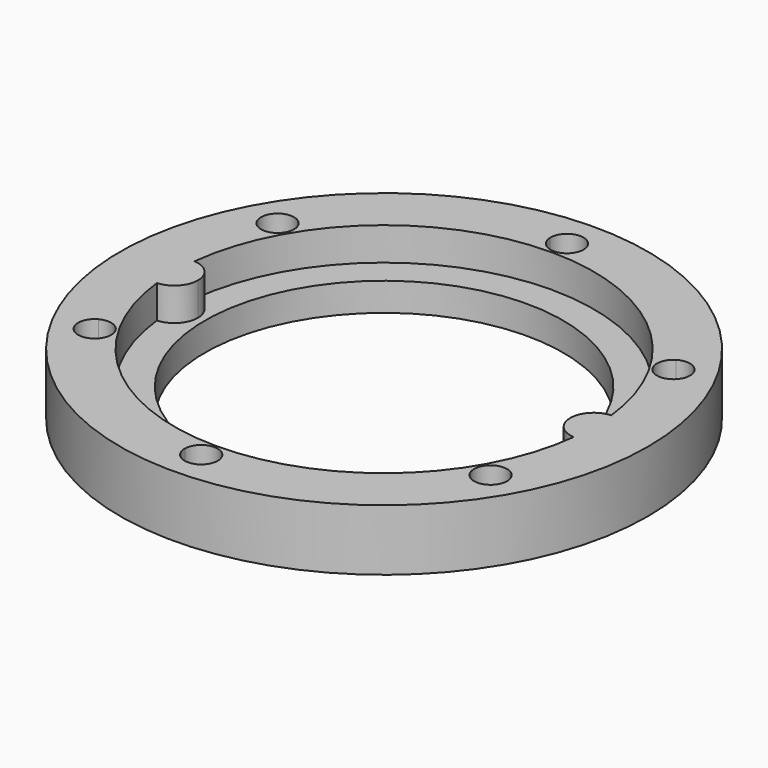
from build123d import *

# Parameters (mm, degrees)
F0_R     = 28
F1_DEPTH = 3.5
F0_R_2   = 19
F2_DEPTH = 3


with BuildPart() as f1:
    # F0 (on Top) → F1 (new body)
    with BuildSketch(Plane.XY):
        Circle(F0_R)
        with BuildLine():
            ThreePointArc((21.8208616615, 10.5788702775), (23.4473621908, 6.1873828305), (24.1994382022, 1.5651487775))
            ThreePointArc((24.1994382022, 1.5651487775), (24.6083464022, 0.8295795605), (24.75, 0))
            ThreePointArc((24.75, 0), (24.6083464022, -0.8295795605), (24.1994382022, -1.5651487775))
            ThreePointArc((24.1994382022, -1.5651487775), (23.4473621908, -6.1873828305), (21.8208616615, -10.5788702775))
            ThreePointArc((21.8208616615, -10.5788702775), (22.5006251005, -11.222795709), (22.7511160418, -12.125))
            ThreePointArc((22.7511160418, -12.125), (21.8486268344, -13.6560863648), (20.0720012344, -13.6079853926))
            ThreePointArc((20.0720012344, -13.6079853926), (12.125, -21.0011160418), (1.7488604271, -24.1868556701))
            ThreePointArc((1.7488604271, -24.1868556701), (1.7497150836, -24.218422694), (1.75, -24.25))
            ThreePointArc((1.75, -24.25), (-0.031577306, -25.9997150836), (-1.7488604271, -24.1868556701))
            ThreePointArc((-1.7488604271, -24.1868556701), (-12.125, -21.0011160418), (-20.0720012344, -13.6079853926))
            ThreePointArc((-20.0720012344, -13.6079853926), (-22.5166604984, -13), (-21.8208616615, -10.5788702775))
            ThreePointArc((-21.8208616615, -10.5788702775), (-23.4473621908, -6.1873828305), (-24.1994382022, -1.5651487775))
            ThreePointArc((-24.1994382022, -1.5651487775), (-24.75, 0), (-24.1994382022, 1.5651487775))
            ThreePointArc((-24.1994382022, 1.5651487775), (-23.4473621908, 6.1873828305), (-21.8208616615, 10.5788702775))
            ThreePointArc((-21.8208616615, 10.5788702775), (-22.5166604984, 13), (-20.0720012344, 13.6079853926))
            ThreePointArc((-20.0720012344, 13.6079853926), (-12.125, 21.0011160418), (-1.7488604271, 24.1868556701))
            ThreePointArc((-1.7488604271, 24.1868556701), (-0.031577306, 25.9997150836), (1.75, 24.25))
            ThreePointArc((1.75, 24.25), (1.7497150836, 24.218422694), (1.7488604271, 24.1868556701))
            ThreePointArc((1.7488604271, 24.1868556701), (12.125, 21.0011160418), (20.0720012344, 13.6079853926))
            ThreePointArc((20.0720012344, 13.6079853926), (21.8486268344, 13.6560863648), (22.7511160418, 12.125))
            ThreePointArc((22.7511160418, 12.125), (22.5006251005, 11.222795709), (21.8208616615, 10.5788702775))
        make_face(mode=Mode.SUBTRACT)
        with BuildLine():
            ThreePointArc((22.1095505618, 2.4960516732), (23.267229147, 2.2836910611), (24.1994382022, 1.5651487775))
            ThreePointArc((24.1994382022, 1.5651487775), (23.4473621908, 6.1873828305), (21.8208616615, 10.5788702775))
            ThreePointArc((21.8208616615, 10.5788702775), (19.4855715851, 11.25), (20.0720012344, 13.6079853926))
            ThreePointArc((20.0720012344, 13.6079853926), (12.125, 21.0011160418), (1.7488604271, 24.1868556701))
            ThreePointArc((1.7488604271, 24.1868556701), (0, 22.5), (-1.7488604271, 24.1868556701))
            ThreePointArc((-1.7488604271, 24.1868556701), (-12.125, 21.0011160418), (-20.0720012344, 13.6079853926))
            ThreePointArc((-20.0720012344, 13.6079853926), (-19.470029677, 12.9725107926), (-19.2511160418, 12.125))
            ThreePointArc((-19.2511160418, 12.125), (-20.0989117508, 10.6254909412), (-21.8208616615, 10.5788702775))
            ThreePointArc((-21.8208616615, 10.5788702775), (-23.4473621908, 6.1873828305), (-24.1994382022, 1.5651487775))
            ThreePointArc((-24.1994382022, 1.5651487775), (-23.267229147, 2.2836910611), (-22.1095505618, 2.4960516732))
            ThreePointArc((-22.1095505618, 2.4960516732), (0, 22.25), (22.1095505618, 2.4960516732))
        make_face()
        with BuildLine():
            ThreePointArc((21.8208616615, -10.5788702775), (23.4473621908, -6.1873828305), (24.1994382022, -1.5651487775))
            ThreePointArc((24.1994382022, -1.5651487775), (23.267229147, -2.2836910611), (22.1095505618, -2.4960516732))
            ThreePointArc((22.1095505618, -2.4960516732), (0, -22.25), (-22.1095505618, -2.4960516732))
            ThreePointArc((-22.1095505618, -2.4960516732), (-23.267229147, -2.2836910611), (-24.1994382022, -1.5651487775))
            ThreePointArc((-24.1994382022, -1.5651487775), (-23.4473621908, -6.1873828305), (-21.8208616615, -10.5788702775))
            ThreePointArc((-21.8208616615, -10.5788702775), (-20.0989117508, -10.6254909412), (-19.2511160418, -12.125))
            ThreePointArc((-19.2511160418, -12.125), (-19.470029677, -12.9725107926), (-20.0720012344, -13.6079853926))
            ThreePointArc((-20.0720012344, -13.6079853926), (-12.125, -21.0011160418), (-1.7488604271, -24.1868556701))
            ThreePointArc((-1.7488604271, -24.1868556701), (0, -22.5), (1.7488604271, -24.1868556701))
            ThreePointArc((1.7488604271, -24.1868556701), (12.125, -21.0011160418), (20.0720012344, -13.6079853926))
            ThreePointArc((20.0720012344, -13.6079853926), (19.4855715851, -11.25), (21.8208616615, -10.5788702775))
        make_face()
        with BuildLine():
            ThreePointArc((22.25, 0), (22.2148598915, 1.25), (22.1095505618, 2.4960516732))
            ThreePointArc((22.1095505618, 2.4960516732), (19.75, 0), (22.1095505618, -2.4960516732))
            ThreePointArc((22.1095505618, -2.4960516732), (22.2148598915, -1.25), (22.25, 0))
        make_face()
        with BuildLine():
            ThreePointArc((-19.75, 0), (-20.4332551644, 1.7173928503), (-22.1095505618, 2.4960516732))
            ThreePointArc((-22.1095505618, 2.4960516732), (-22.25, 0), (-22.1095505618, -2.4960516732))
            ThreePointArc((-22.1095505618, -2.4960516732), (-20.4332551644, -1.7173928503), (-19.75, 0))
        make_face()
        with BuildLine():
            ThreePointArc((24.1994382022, -1.5651487775), (24.2373562544, -0.7829826293), (24.25, 0))
            ThreePointArc((24.25, 0), (24.2373562544, 0.7829826293), (24.1994382022, 1.5651487775))
            ThreePointArc((24.1994382022, 1.5651487775), (23.267229147, 2.2836910611), (22.1095505618, 2.4960516732))
            ThreePointArc((22.1095505618, 2.4960516732), (22.2148598915, 1.25), (22.25, 0))
            ThreePointArc((22.25, 0), (22.2148598915, -1.25), (22.1095505618, -2.4960516732))
            ThreePointArc((22.1095505618, -2.4960516732), (23.267229147, -2.2836910611), (24.1994382022, -1.5651487775))
        make_face()
        with BuildLine():
            ThreePointArc((-22.1095505618, -2.4960516732), (-22.25, 0), (-22.1095505618, 2.4960516732))
            ThreePointArc((-22.1095505618, 2.4960516732), (-23.267229147, 2.2836910611), (-24.1994382022, 1.5651487775))
            ThreePointArc((-24.1994382022, 1.5651487775), (-24.25, 0), (-24.1994382022, -1.5651487775))
            ThreePointArc((-24.1994382022, -1.5651487775), (-23.267229147, -2.2836910611), (-22.1095505618, -2.4960516732))
        make_face()
        with BuildLine():
            ThreePointArc((24.1994382022, 1.5651487775), (24.2373562544, 0.7829826293), (24.25, 0))
            ThreePointArc((24.25, 0), (24.2373562544, -0.7829826293), (24.1994382022, -1.5651487775))
            ThreePointArc((24.1994382022, -1.5651487775), (24.6083464022, -0.8295795605), (24.75, 0))
            ThreePointArc((24.75, 0), (24.6083464022, 0.8295795605), (24.1994382022, 1.5651487775))
        make_face()
        with BuildLine():
            ThreePointArc((-24.1994382022, -1.5651487775), (-24.25, 0), (-24.1994382022, 1.5651487775))
            ThreePointArc((-24.1994382022, 1.5651487775), (-24.75, 0), (-24.1994382022, -1.5651487775))
        make_face()
    extrude(amount=F1_DEPTH)

    # F0 (on Top) → F2 (join)
    with BuildSketch(Plane.XY):
        Circle(F0_R)
        with BuildLine():
            ThreePointArc((21.8208616615, 10.5788702775), (23.4473621908, 6.1873828305), (24.1994382022, 1.5651487775))
            ThreePointArc((24.1994382022, 1.5651487775), (24.6083464022, 0.8295795605), (24.75, 0))
            ThreePointArc((24.75, 0), (24.6083464022, -0.8295795605), (24.1994382022, -1.5651487775))
            ThreePointArc((24.1994382022, -1.5651487775), (23.4473621908, -6.1873828305), (21.8208616615, -10.5788702775))
            ThreePointArc((21.8208616615, -10.5788702775), (22.5006251005, -11.222795709), (22.7511160418, -12.125))
            ThreePointArc((22.7511160418, -12.125), (21.8486268344, -13.6560863648), (20.0720012344, -13.6079853926))
            ThreePointArc((20.0720012344, -13.6079853926), (12.125, -21.0011160418), (1.7488604271, -24.1868556701))
            ThreePointArc((1.7488604271, -24.1868556701), (1.7497150836, -24.218422694), (1.75, -24.25))
            ThreePointArc((1.75, -24.25), (-0.031577306, -25.9997150836), (-1.7488604271, -24.1868556701))
            ThreePointArc((-1.7488604271, -24.1868556701), (-12.125, -21.0011160418), (-20.0720012344, -13.6079853926))
            ThreePointArc((-20.0720012344, -13.6079853926), (-22.5166604984, -13), (-21.8208616615, -10.5788702775))
            ThreePointArc((-21.8208616615, -10.5788702775), (-23.4473621908, -6.1873828305), (-24.1994382022, -1.5651487775))
            ThreePointArc((-24.1994382022, -1.5651487775), (-24.75, 0), (-24.1994382022, 1.5651487775))
            ThreePointArc((-24.1994382022, 1.5651487775), (-23.4473621908, 6.1873828305), (-21.8208616615, 10.5788702775))
            ThreePointArc((-21.8208616615, 10.5788702775), (-22.5166604984, 13), (-20.0720012344, 13.6079853926))
            ThreePointArc((-20.0720012344, 13.6079853926), (-12.125, 21.0011160418), (-1.7488604271, 24.1868556701))
            ThreePointArc((-1.7488604271, 24.1868556701), (-0.031577306, 25.9997150836), (1.75, 24.25))
            ThreePointArc((1.75, 24.25), (1.7497150836, 24.218422694), (1.7488604271, 24.1868556701))
            ThreePointArc((1.7488604271, 24.1868556701), (12.125, 21.0011160418), (20.0720012344, 13.6079853926))
            ThreePointArc((20.0720012344, 13.6079853926), (21.8486268344, 13.6560863648), (22.7511160418, 12.125))
            ThreePointArc((22.7511160418, 12.125), (22.5006251005, 11.222795709), (21.8208616615, 10.5788702775))
        make_face(mode=Mode.SUBTRACT)
        with BuildLine():
            ThreePointArc((22.1095505618, -2.4960516732), (19.75, 0), (22.1095505618, 2.4960516732))
            ThreePointArc((22.1095505618, 2.4960516732), (0, 22.25), (-22.1095505618, 2.4960516732))
            ThreePointArc((-22.1095505618, 2.4960516732), (-20.4332551644, 1.7173928503), (-19.75, 0))
            ThreePointArc((-19.75, 0), (-20.4332551644, -1.7173928503), (-22.1095505618, -2.4960516732))
            ThreePointArc((-22.1095505618, -2.4960516732), (0, -22.25), (22.1095505618, -2.4960516732))
        make_face()
        Circle(F0_R_2, mode=Mode.SUBTRACT)
        with BuildLine():
            ThreePointArc((22.1095505618, 2.4960516732), (23.267229147, 2.2836910611), (24.1994382022, 1.5651487775))
            ThreePointArc((24.1994382022, 1.5651487775), (23.4473621908, 6.1873828305), (21.8208616615, 10.5788702775))
            ThreePointArc((21.8208616615, 10.5788702775), (19.4855715851, 11.25), (20.0720012344, 13.6079853926))
            ThreePointArc((20.0720012344, 13.6079853926), (12.125, 21.0011160418), (1.7488604271, 24.1868556701))
            ThreePointArc((1.7488604271, 24.1868556701), (0, 22.5), (-1.7488604271, 24.1868556701))
            ThreePointArc((-1.7488604271, 24.1868556701), (-12.125, 21.0011160418), (-20.0720012344, 13.6079853926))
            ThreePointArc((-20.0720012344, 13.6079853926), (-19.470029677, 12.9725107926), (-19.2511160418, 12.125))
            ThreePointArc((-19.2511160418, 12.125), (-20.0989117508, 10.6254909412), (-21.8208616615, 10.5788702775))
            ThreePointArc((-21.8208616615, 10.5788702775), (-23.4473621908, 6.1873828305), (-24.1994382022, 1.5651487775))
            ThreePointArc((-24.1994382022, 1.5651487775), (-23.267229147, 2.2836910611), (-22.1095505618, 2.4960516732))
            ThreePointArc((-22.1095505618, 2.4960516732), (0, 22.25), (22.1095505618, 2.4960516732))
        make_face()
        with BuildLine():
            ThreePointArc((21.8208616615, -10.5788702775), (23.4473621908, -6.1873828305), (24.1994382022, -1.5651487775))
            ThreePointArc((24.1994382022, -1.5651487775), (23.267229147, -2.2836910611), (22.1095505618, -2.4960516732))
            ThreePointArc((22.1095505618, -2.4960516732), (0, -22.25), (-22.1095505618, -2.4960516732))
            ThreePointArc((-22.1095505618, -2.4960516732), (-23.267229147, -2.2836910611), (-24.1994382022, -1.5651487775))
            ThreePointArc((-24.1994382022, -1.5651487775), (-23.4473621908, -6.1873828305), (-21.8208616615, -10.5788702775))
            ThreePointArc((-21.8208616615, -10.5788702775), (-20.0989117508, -10.6254909412), (-19.2511160418, -12.125))
            ThreePointArc((-19.2511160418, -12.125), (-19.470029677, -12.9725107926), (-20.0720012344, -13.6079853926))
            ThreePointArc((-20.0720012344, -13.6079853926), (-12.125, -21.0011160418), (-1.7488604271, -24.1868556701))
            ThreePointArc((-1.7488604271, -24.1868556701), (0, -22.5), (1.7488604271, -24.1868556701))
            ThreePointArc((1.7488604271, -24.1868556701), (12.125, -21.0011160418), (20.0720012344, -13.6079853926))
            ThreePointArc((20.0720012344, -13.6079853926), (19.4855715851, -11.25), (21.8208616615, -10.5788702775))
        make_face()
        with BuildLine():
            ThreePointArc((22.25, 0), (22.2148598915, 1.25), (22.1095505618, 2.4960516732))
            ThreePointArc((22.1095505618, 2.4960516732), (19.75, 0), (22.1095505618, -2.4960516732))
            ThreePointArc((22.1095505618, -2.4960516732), (22.2148598915, -1.25), (22.25, 0))
        make_face()
        with BuildLine():
            ThreePointArc((-19.75, 0), (-20.4332551644, 1.7173928503), (-22.1095505618, 2.4960516732))
            ThreePointArc((-22.1095505618, 2.4960516732), (-22.25, 0), (-22.1095505618, -2.4960516732))
            ThreePointArc((-22.1095505618, -2.4960516732), (-20.4332551644, -1.7173928503), (-19.75, 0))
        make_face()
        with BuildLine():
            ThreePointArc((24.1994382022, -1.5651487775), (24.2373562544, -0.7829826293), (24.25, 0))
            ThreePointArc((24.25, 0), (24.2373562544, 0.7829826293), (24.1994382022, 1.5651487775))
            ThreePointArc((24.1994382022, 1.5651487775), (23.267229147, 2.2836910611), (22.1095505618, 2.4960516732))
            ThreePointArc((22.1095505618, 2.4960516732), (22.2148598915, 1.25), (22.25, 0))
            ThreePointArc((22.25, 0), (22.2148598915, -1.25), (22.1095505618, -2.4960516732))
            ThreePointArc((22.1095505618, -2.4960516732), (23.267229147, -2.2836910611), (24.1994382022, -1.5651487775))
        make_face()
        with BuildLine():
            ThreePointArc((-22.1095505618, -2.4960516732), (-22.25, 0), (-22.1095505618, 2.4960516732))
            ThreePointArc((-22.1095505618, 2.4960516732), (-23.267229147, 2.2836910611), (-24.1994382022, 1.5651487775))
            ThreePointArc((-24.1994382022, 1.5651487775), (-24.25, 0), (-24.1994382022, -1.5651487775))
            ThreePointArc((-24.1994382022, -1.5651487775), (-23.267229147, -2.2836910611), (-22.1095505618, -2.4960516732))
        make_face()
        with BuildLine():
            ThreePointArc((24.1994382022, 1.5651487775), (24.2373562544, 0.7829826293), (24.25, 0))
            ThreePointArc((24.25, 0), (24.2373562544, -0.7829826293), (24.1994382022, -1.5651487775))
            ThreePointArc((24.1994382022, -1.5651487775), (24.6083464022, -0.8295795605), (24.75, 0))
            ThreePointArc((24.75, 0), (24.6083464022, 0.8295795605), (24.1994382022, 1.5651487775))
        make_face()
        with BuildLine():
            ThreePointArc((-24.1994382022, -1.5651487775), (-24.25, 0), (-24.1994382022, 1.5651487775))
            ThreePointArc((-24.1994382022, 1.5651487775), (-24.75, 0), (-24.1994382022, -1.5651487775))
        make_face()
    extrude(amount=-F2_DEPTH)


solid = f1.part
